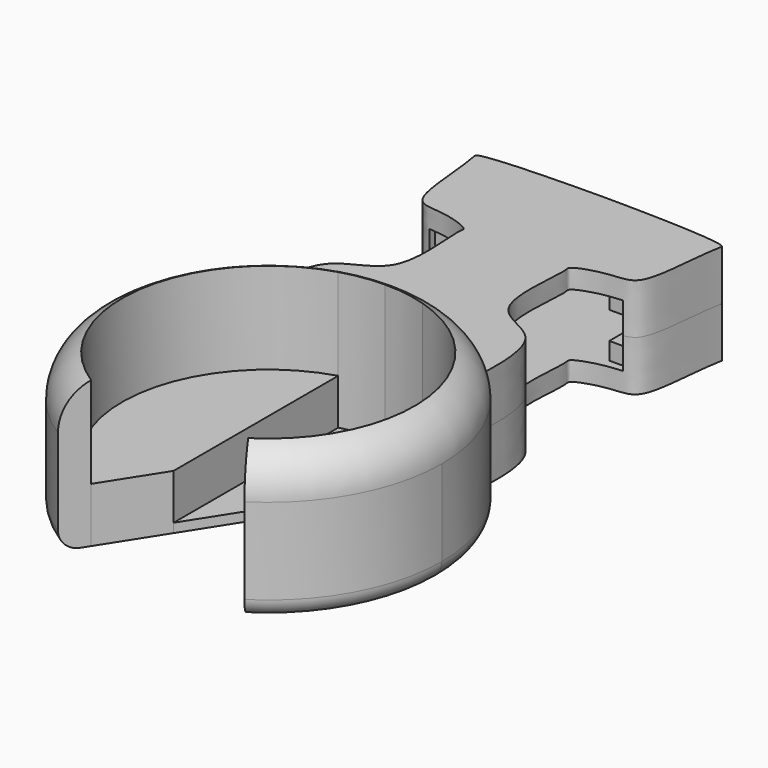
from build123d import *

# Parameters (mm, degrees)
F1_DEPTH    = 1
F2_DEPTH    = 6
F3_DEPTH    = 16
F5_T2_ANGLE = 359.64
F6_R        = 2
F10_DEPTH   = 5.5
F13_W       = 21.2
F13_H       = 6.8
F14_DEPTH   = 27
F16_W       = 2.1
F16_H       = 1.9
F17_DEPTH   = 4


# Not quite as in the source:
# - a fillet or chamfer that OpenCascade refuses, or shapes differently, is made with other operations: its cross-section is extruded or revolved along the edge and cut away or added


with BuildPart() as f1:
    # F0 (on Top) → F1 (new body)
    with BuildSketch(Plane.XY):
        with BuildLine():
            Line((4.6, -7.2205536547), (4.6, 15.3244902036))
            ThreePointArc((4.6, 15.3244902036), (2.3246673679, 15.8302217808), (0, 16))
            ThreePointArc((0, 16), (-2.3246673679, 15.8302217808), (-4.6, 15.3244902036))
            Line((-4.6, 15.3244902036), (-4.6, -7.2205536547))
            Line((-4.6, -7.2205536547), (0, 0))
            Line((0, 0), (4.6, -7.2205536547))
        make_face()
    extrude(amount=F1_DEPTH)

    # F0 (on Top) → F2 (join)
    with BuildSketch(Plane.XY):
        with BuildLine():
            ThreePointArc((8.5967937335, -13.494263133), (14.0276280913, -7.6958203027), (16, 0))
            ThreePointArc((16, 0), (12.8374452287, 9.5498691091), (4.6, 15.3244902036))
            Line((4.6, 15.3244902036), (4.6, -7.2205536547))
            Line((4.6, -7.2205536547), (8.5967937335, -13.494263133))
        make_face()
        with BuildLine():
            Line((-4.6, -7.2205536547), (-4.6, 15.3244902036))
            ThreePointArc((-4.6, 15.3244902036), (-15.848311493, 2.1979587848), (-8.5967937335, -13.494263133))
            Line((-8.5967937335, -13.494263133), (-4.6, -7.2205536547))
        make_face()
    extrude(amount=F2_DEPTH)

    # F0 (on Top) → F3 (join)
    with BuildSketch(Plane.XY):
        with BuildLine():
            ThreePointArc((-4.6, 15.3244902036), (-2.3246673679, 15.8302217808), (0, 16))
            Line((0, 16), (-4.6, 16))
            Line((-4.6, 16), (-4.6, 15.3244902036))
        make_face()
        with BuildLine():
            ThreePointArc((0, 16), (2.3246673679, 15.8302217808), (4.6, 15.3244902036))
            Line((4.6, 15.3244902036), (4.6, 16))
            Line((4.6, 16), (0, 16))
        make_face()
        with BuildLine():
            ThreePointArc((4.6, 15.3244902036), (12.8374452287, 9.5498691091), (16, 0))
            ThreePointArc((16, 0), (14.0276280913, -7.6958203027), (8.5967937335, -13.494263133))
            Line((8.5967937335, -13.494263133), (10.2086925586, -16.0244374704))
            ThreePointArc((10.2086925586, -16.0244374704), (16.6578083584, -9.1387866095), (19, 0))
            ThreePointArc((19, 0), (-9.1387866095, 16.6578083584), (-10.2086925586, -16.0244374704))
            Line((-10.2086925586, -16.0244374704), (-8.5967937335, -13.494263133))
            ThreePointArc((-8.5967937335, -13.494263133), (-15.848311493, 2.1979587848), (-4.6, 15.3244902036))
            Line((-4.6, 15.3244902036), (-4.6, 16))
            Line((-4.6, 16), (0, 16))
            Line((0, 16), (4.6, 16))
            Line((4.6, 16), (4.6, 15.3244902036))
        make_face()
    extrude(amount=F3_DEPTH)

    # F5: fillet of radius 5 on 1 edges, made by hand

    # F5_s1 → F5_t2 (revolve, cut)
    with BuildSketch(Plane(origin=(0, 0, 0), x_dir=(0, 0, 1), z_dir=(-0.9999950652, -0.0031415875, 0))):
        with BuildLine():
            ThreePointArc((11.417424305, -19), (14.1560370926, -18.1833001327), (16, -16))
            Line((16, -16), (16, -19))
            Line((16, -19), (11.417424305, -19))
        make_face()
    revolve(axis=Axis((0, 0, 16), (0, 0, 1)), revolution_arc=F5_T2_ANGLE, mode=Mode.SUBTRACT)

    # F6
    f6_edges = [f1.edges().sort_by_distance(p)[0] for p in [
        (0, 19, 0),
    ]]
    fillet(f6_edges, radius=F6_R)

    # F9 (on offset) → F10 (join, symmetric)
    with BuildSketch(Plane.XY.offset(6.7)):
        with BuildLine():
            Line((12.1534438804, 12.4591999873), (12.1534438804, 13.2602723315))
            add(Edge.make_bspline(
                [(12.1534438804, 13.2602723315), (12.2485305409, 15.5137947327), (12.6472970261, 22.9116892126), (4.4309754502, 23.3856485338), (6.1277558694, 33.2017689451), (5.4340440691, 34.1607702042), (9.2573649007, 35.4222833934), (13.0166322284, 34.9603355308), (12.8244706572, 41.5928681515), (13.5, 45.1432300031)],
                knots=[0, 0, 0, 0, 0.1834261886, 0.3390540854, 0.5215473334, 0.5780460819, 0.6966579264, 0.8049708304, 1, 1, 1, 1], degree=3))
            add(Edge.make_bspline(
                [(13.5, 45.1432300031), (13.7662592158, 45.9176948786), (2.9332311824, 46.0396686256), (0, 46.0432300031)],
                knots=[0, 0, 0, 0, 13.5299667405, 13.5299667405, 13.5299667405, 13.5299667405], degree=3))
            add(Edge.make_bspline(
                [(-13.5, 45.1432300031), (-13.7662592158, 45.9176948786), (-2.9332311824, 46.0396686256), (0, 46.0432300031)],
                knots=[0, 0, 0, 0, 13.5299667405, 13.5299667405, 13.5299667405, 13.5299667405], degree=3))
            add(Edge.make_bspline(
                [(-12.1534438804, 13.2602723315), (-12.2485305409, 15.5137947327), (-12.6472970261, 22.9116892126), (-4.4309754502, 23.3856485338), (-6.1277558694, 33.2017689451), (-5.4340440691, 34.1607702042), (-9.2573649007, 35.4222833934), (-13.0166322284, 34.9603355308), (-12.8244706572, 41.5928681515), (-13.5, 45.1432300031)],
                knots=[0, 0, 0, 0, 0.1834261886, 0.3390540854, 0.5215473334, 0.5780460819, 0.6966579264, 0.8049708304, 1, 1, 1, 1], degree=3))
            Line((-12.1534438804, 13.2602723315), (-12.1534438804, 12.4591999873))
            Line((-12.1534438804, 12.4591999873), (0, 18.0332660675))
            Line((0, 18.0332660675), (12.1534438804, 12.4591999873))
        make_face()
    extrude(amount=F10_DEPTH, both=True)

    # F13 (on plane+point) → F14 (cut)
    with BuildSketch(Plane.XZ.offset(-46.0432300031)):
        with Locations((0, 6.7)):
            Rectangle(F13_W, F13_H)
    extrude(amount=F14_DEPTH, mode=Mode.SUBTRACT)

    # F16 (on offset) → F17 (join)
    with BuildSketch(Plane.XZ.offset(-36.0432300031)):
        with Locations((-9.55, 4.25)):
            Rectangle(F16_W, F16_H)
        with Locations((-9.55, 9.15)):
            Rectangle(F16_W, F16_H)
        with Locations((9.55, 9.15)):
            Rectangle(F16_W, F16_H)
        with Locations((9.55, 4.25)):
            Rectangle(F16_W, F16_H)
    extrude(amount=-F17_DEPTH)


solid = f1.part
